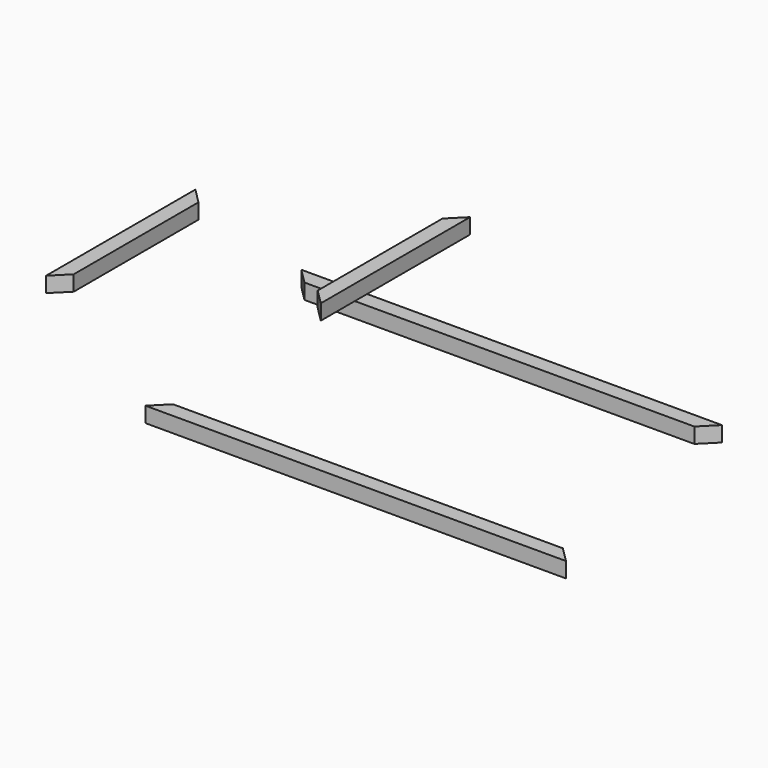
from build123d import *

# Parameters (mm, degrees)
F0_W      = 30
F0_H      = 30
F1_DEPTH  = 822
F2_W      = 30
F2_H      = 30
F3_DEPTH  = 364.8
F4_W      = 30
F4_H      = 30
F5_DEPTH  = 822
F6_W      = 30
F6_H      = 30
F7_DEPTH  = 364.8
F8_SIZE   = 29.99999
F8_2_SIZE = 29.99999
F8_3_SIZE = 29.99999
F8_4_SIZE = 29.99999


# Not quite as in the source:
# - a fillet or chamfer is up to 0.001 mm smaller than in the source, because OpenCascade refuses the exact size


with BuildPart() as f1:
    # F0 (on Right) → F1 (new body)
    with BuildSketch(Plane.YZ):
        with Locations((-43.334082365, -270.7813239098)):
            Rectangle(F0_W, F0_H)
    extrude(amount=F1_DEPTH)

    # F8#4 (size 30 in the source; OpenCascade refuses exactly that, so slightly less here)
    f8_4_edges = [f1.edges().sort_by_distance(p)[0] for p in [
        (822, -58.334082, -270.781324),
        (0, -58.334082, -270.781324),
    ]]
    chamfer(f8_4_edges, length=F8_4_SIZE)


with BuildPart() as f3:
    # F2 (on Front) → F3 (new body)
    with BuildSketch(Plane.XZ):
        with Locations((-214.8419408661, -219.0126031637)):
            Rectangle(F2_W, F2_H)
    extrude(amount=F3_DEPTH)

    # F8#2 (size 30 in the source; OpenCascade refuses exactly that, so slightly less here)
    f8_2_edges = [f3.edges().sort_by_distance(p)[0] for p in [
        (-199.841941, 0, -219.012603),
        (-199.841941, -364.8, -219.012603),
    ]]
    chamfer(f8_2_edges, length=F8_2_SIZE)


with BuildPart() as f5:
    # F4 (on Right) → F5 (new body)
    with BuildSketch(Plane.YZ):
        with Locations((-394.3848624069, -349.8105704784)):
            Rectangle(F4_W, F4_H)
    extrude(amount=F5_DEPTH)

    # F8#3 (size 30 in the source; OpenCascade refuses exactly that, so slightly less here)
    f8_3_edges = [f5.edges().sort_by_distance(p)[0] for p in [
        (0, -379.384862, -349.81057),
        (822, -379.384862, -349.81057),
    ]]
    chamfer(f8_3_edges, length=F8_3_SIZE)


with BuildPart() as f7:
    # F6 (on Front) → F7 (new body)
    with BuildSketch(Plane.XZ):
        with Locations((292.1046539125, -91.8692350388)):
            Rectangle(F6_W, F6_H)
    extrude(amount=F7_DEPTH)

    # F8 (size 30 in the source; OpenCascade refuses exactly that, so slightly less here)
    f8_edges = [f7.edges().sort_by_distance(p)[0] for p in [
        (277.104654, 0, -91.869235),
        (277.104654, -364.8, -91.869235),
    ]]
    chamfer(f8_edges, length=F8_SIZE)


solid = Compound([f1.part, f3.part, f5.part, f7.part])
